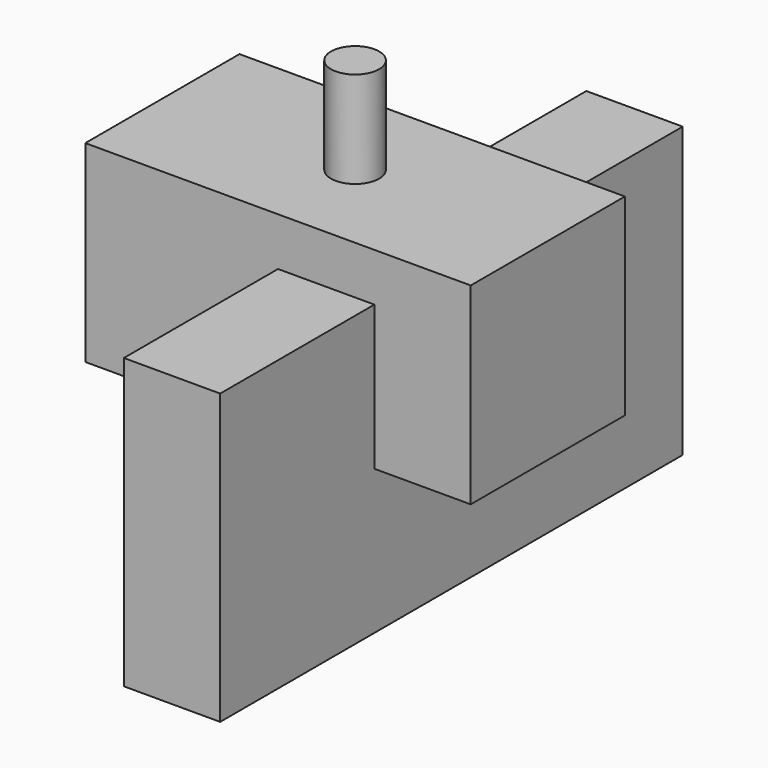
from build123d import *

# Parameters (mm, degrees)
F0_W     = 50.8
F0_H     = 25.4
F1_DEPTH = 25.4
F2_R     = 3.175
F3_DEPTH = 12.7
F4_W     = 76.2
F4_H     = 38.1
F5_DEPTH = 12.7
F6_R     = 6.35
F7_DEPTH = 38.101


with BuildPart() as f1:
    # F0 (on Top) → F1 (new body)
    with BuildSketch(Plane.XY):
        Rectangle(F0_W, F0_H)
    extrude(amount=F1_DEPTH)

    # F2 (on face) → F3 (join)
    with BuildSketch(Plane.XY.offset(25.4)):
        Circle(F2_R)
    extrude(amount=F3_DEPTH)


with BuildPart() as f5:
    # F4 (on Right) → F5 (new body)
    with BuildSketch(Plane.YZ):
        Rectangle(F4_W, F4_H)
    extrude(amount=F5_DEPTH)

    # F6 (on face) → F7 (cut, through all)
    with BuildSketch(Plane.YZ.offset(12.7)):
        Circle(F6_R)
    extrude(amount=-F7_DEPTH, mode=Mode.SUBTRACT)


solid = Compound([f1.part, f5.part])
